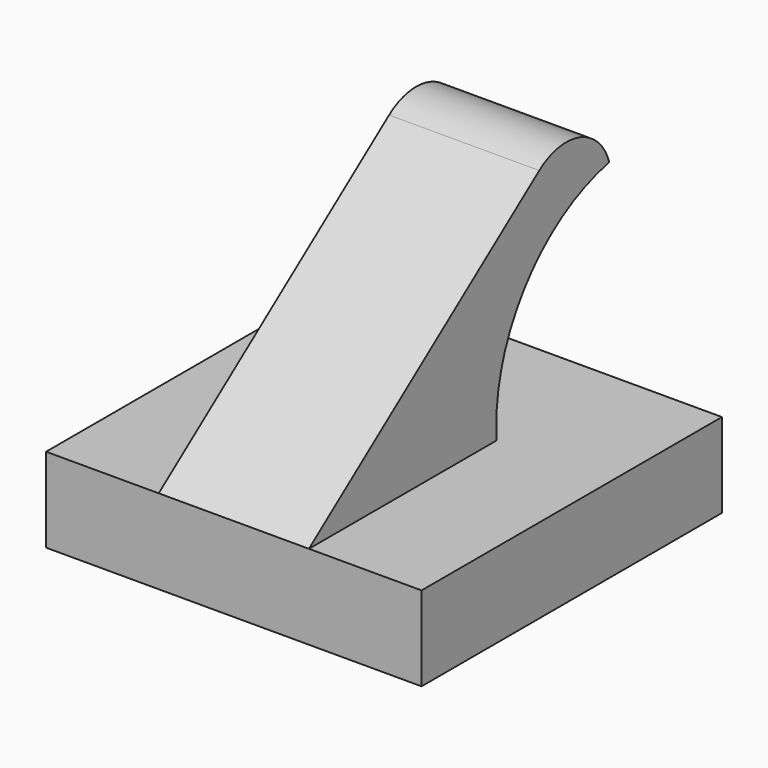
from build123d import *

# Parameters (mm, degrees)
F1_DEPTH    = 20
F2_W        = 6
F2_H        = 15
F3_DEPTH    = 20.001
F4_T1_DEPTH = 37.1421356237
F5_W        = 20
F5_H        = 20
F5_W_2      = 18
F5_H_2      = 18
F6_DEPTH    = 1.5


# Not quite as in the source:
# - a fillet or chamfer that OpenCascade refuses, or shapes differently, is made with other operations: its cross-section is extruded or revolved along the edge and cut away or added


with BuildPart() as f1:
    # F0 (on Right) → F1 (new body)
    with BuildSketch(Plane.YZ):
        with BuildLine():
            Line((-18.178238757, 7.9620768987), (-18.178238757, 4.9620768987))
            Line((-18.178238757, 4.9620768987), (1.821761243, 4.9620768987))
            Line((1.821761243, 4.9620768987), (1.821761243, 7.9620768987))
            Line((1.821761243, 7.9620768987), (-5.678238757, 7.9620768987))
            Line((-5.678238757, 7.9620768987), (-5.678238757, 9.3611253762))
            ThreePointArc((-5.678238757, 9.3611253762), (-5.2512465802, 11.5609410366), (-4.321354907, 13.5997673497))
            ThreePointArc((-4.321354907, 13.5997673497), (-1.7002475397, 16.4152583597), (1.821761243, 17.9620768987))
            Line((1.821761243, 17.9620768987), (1.821761243, 22.9620768987))
            Line((1.821761243, 22.9620768987), (-18.178238757, 7.9620768987))
        make_face()
    extrude(amount=F1_DEPTH)

    # F2 (on face) → F3 (cut, through all)
    with BuildSketch(Plane(origin=(0, 1.821761243, 0), x_dir=(-1, 0, 0), z_dir=(0, 1, 0))):
        with Locations((-17, 15.4620768987)):
            Rectangle(F2_W, F2_H)
        with Locations((-3, 15.4620768987)):
            Rectangle(F2_W, F2_H)
    extrude(amount=-F3_DEPTH, mode=Mode.SUBTRACT)

    # F4: fillet of radius 3 on 1 edges, made by hand

    # F4_s2 → F4_t1 (cut)
    with BuildSketch(Plane.YZ.offset(-8.5710678119)):
        with BuildLine():
            ThreePointArc((-2.8409804568, 19.4650206238), (-0.1206191471, 19.9203551155), (1.821761243, 17.9620768987))
            Line((1.821761243, 17.9620768987), (1.821761243, 22.9620768987))
            Line((1.821761243, 22.9620768987), (-2.8409804568, 19.4650206238))
        make_face()
    extrude(amount=F4_T1_DEPTH, mode=Mode.SUBTRACT)

    # F5 (on face) → F6 (join)
    with BuildSketch(Plane(origin=(0, 0, 4.9620768987), x_dir=(1, 0, 0), z_dir=(0, 0, -1))):
        with Locations((10, 8.178238757)):
            Rectangle(F5_W, F5_H)
        with Locations((10, 8.178238757)):
            Rectangle(F5_W_2, F5_H_2, mode=Mode.SUBTRACT)
    extrude(amount=F6_DEPTH)


solid = f1.part
